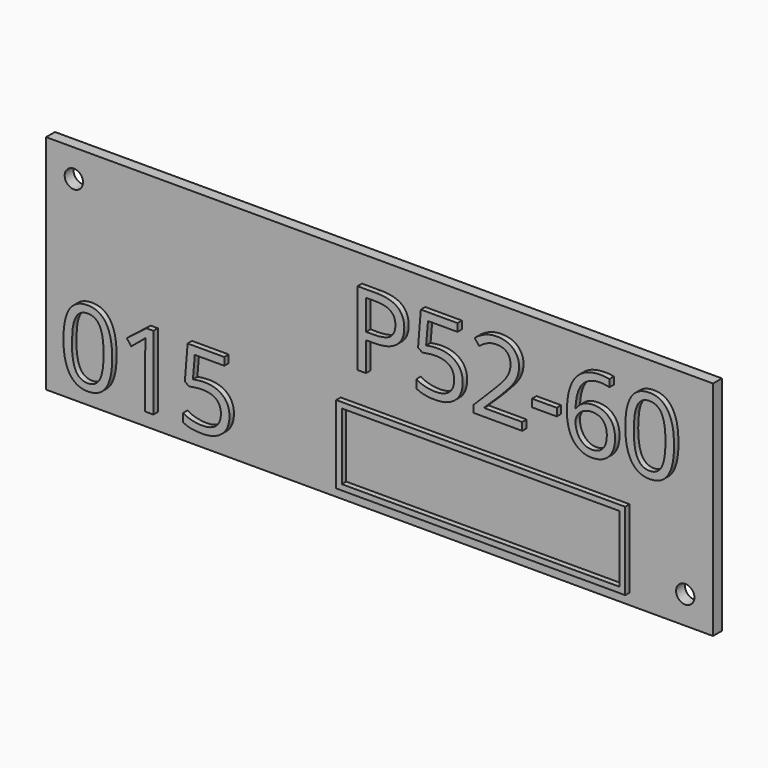
from build123d import *

# Parameters (mm, degrees)
F0_W         = 120
F0_H         = 40
F1_DEPTH     = 2
F3_D         = 3.3
F4_TEXT_SIZE = 18.6001453136
F5_DEPTH     = 1
F6_TEXT_SIZE = 18.5776487663
F7_DEPTH     = 1
F8_W         = 52
F8_H         = 14
F8_W_2       = 49.99999962
F8_H_2       = 11.99999962
F9_DEPTH     = 1


# Not quite as in the source:
# - Text() gives the source's letters only with a copy of the font that has no kerning and outlines rounded to 1/6400 em; it was checked with that copy


with BuildPart() as f1:
    # F0 (on Front) → F1 (new body)
    with BuildSketch(Plane.XZ):
        Rectangle(F0_W, F0_H)
    extrude(amount=F1_DEPTH)

    # F3 (through all)
    with Locations(Plane.XZ.offset(2)):
        with Locations((-55, 15), (55, -15)):
            Hole(F3_D / 2)

    # F4 (on face) → F5 (join)
    with BuildSketch(Plane.XZ.offset(2)):
        with Locations((-5, 2)):
            Text('P52-60', F4_TEXT_SIZE, font='Open Sans', text_align=(TextAlign.LEFT, TextAlign.BOTTOM))
    extrude(amount=F5_DEPTH)

    # F6 (on face) → F7 (join)
    with BuildSketch(Plane.XZ.offset(2)):
        with Locations((-57, -17)):
            Text('015', F6_TEXT_SIZE, font='Open Sans', text_align=(TextAlign.LEFT, TextAlign.BOTTOM))
    extrude(amount=F7_DEPTH)

    # F8 (on face) → F9 (join)
    with BuildSketch(Plane.XZ.offset(2)):
        with Locations((19, -11)):
            Rectangle(F8_W, F8_H)
        with Locations((19, -11)):
            Rectangle(F8_W_2, F8_H_2, mode=Mode.SUBTRACT)
    extrude(amount=F9_DEPTH)


solid = f1.part
